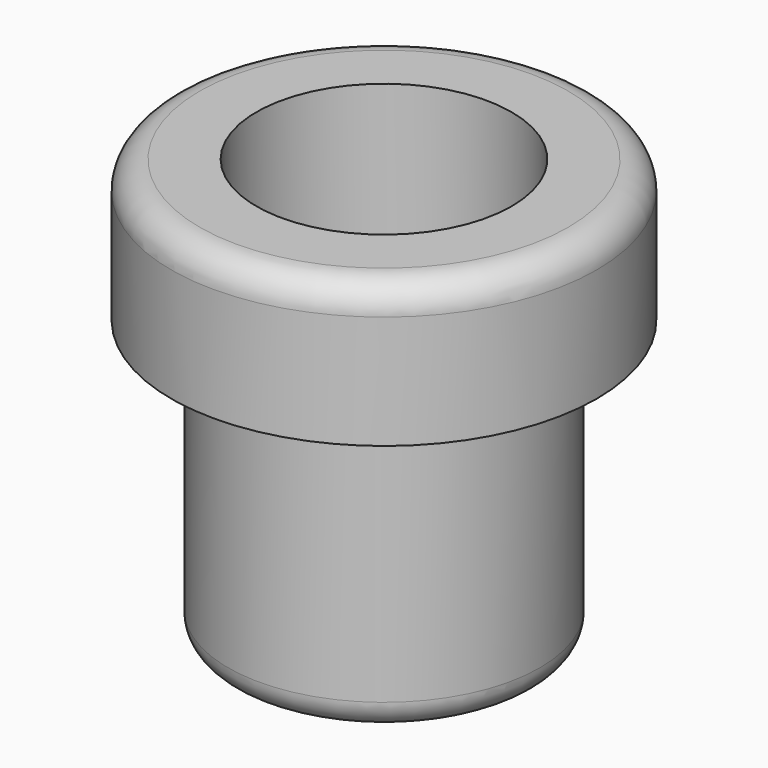
from build123d import *

# Parameters (mm, degrees)
F0_R     = 5.5
F0_R_2   = 4.5
F1_DEPTH = 15
F0_R_3   = 7.5
F2_DEPTH = 5
F3_R     = 0.99999


# Not quite as in the source:
# - a fillet or chamfer is up to 0.001 mm smaller than in the source, because OpenCascade refuses the exact size


with BuildPart() as f1:
    # F0 (on Top) → F1 (new body)
    with BuildSketch(Plane.XY):
        Circle(F0_R)
        Circle(F0_R_2, mode=Mode.SUBTRACT)
    extrude(amount=-F1_DEPTH)

    # F0 (on Top) → F2 (join)
    with BuildSketch(Plane.XY):
        Circle(F0_R_3)
        Circle(F0_R, mode=Mode.SUBTRACT)
    extrude(amount=-F2_DEPTH)

    # F3 (radius 1 in the source; OpenCascade refuses exactly that, so slightly less here)
    f3_edges = [f1.edges().sort_by_distance(p)[0] for p in [
        (-7.5, 0, 0),
        (-5.5, 0, -15),
    ]]
    fillet(f3_edges, radius=F3_R)


solid = f1.part
